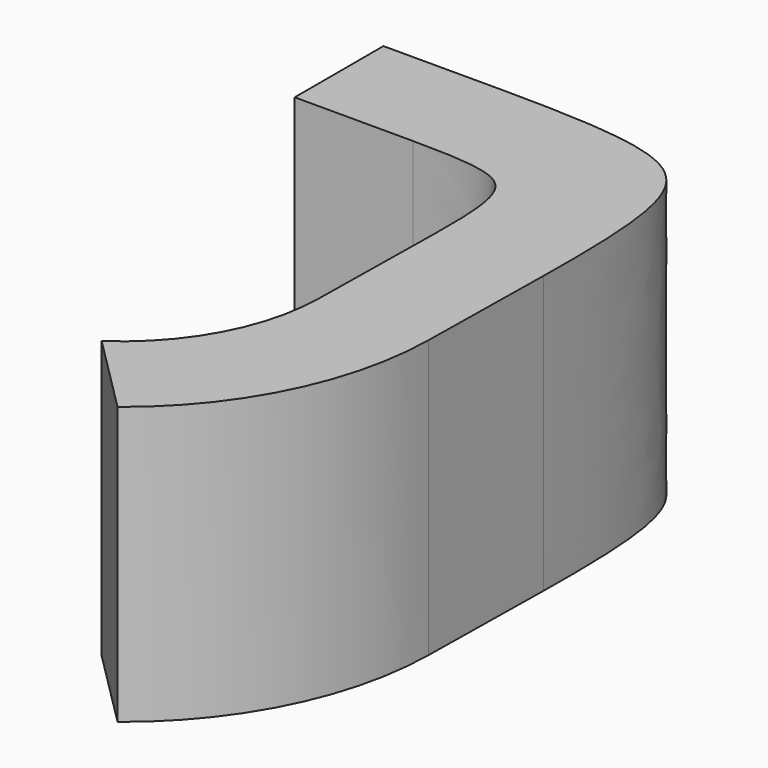
from build123d import *

# Parameters (mm, degrees)
F3_DEPTH    = 5
F4_T1_DEPTH = 5
F5_T1_DEPTH = 25.3094755674


# Not quite as in the source:
# - a fillet or chamfer that OpenCascade refuses, or shapes differently, is made with other operations: its cross-section is extruded or revolved along the edge and cut away or added
# - a feature of the source that left no trace in its solid (it failed there, or was rolled back) is left out


with BuildPart() as f3:
    # F2 (on Top) → F3 (new body)
    with BuildSketch(Plane.XY):
        with BuildLine():
            Line((5.5017601699, 0), (5.5017601699, -2))
            Line((5.5017601699, -2), (9.6698484997, -2))
            Line((9.6698484997, -2), (9.5995756294, -6.5762830432))
            ThreePointArc((9.5995756294, -6.5762830432), (9.167895168, -8.2311078505), (8.0212889249, -9.5))
            Line((8.0212889249, -9.5), (9.4518866721, -10.9305977473))
            ThreePointArc((9.4518866721, -10.9305977473), (11.0154330705, -9.0120786534), (11.5993398679, -6.6069911903))
            Line((11.5993398679, -6.6069911903), (11.7007960564, 0))
            Line((11.7007960564, 0), (5.5017601699, 0))
        make_face()
    extrude(amount=F3_DEPTH)

    # F4: fillet of radius 2 on 1 edges, made by hand

    # F4_s2 → F4_t1 (join)
    with BuildSketch(Plane.XY):
        with BuildLine():
            add(Edge.make_bspline(
                [(7.638900943, -2), (9.6698484997, -2), (9.6386651815, -4.0307081471)],
                knots=[0, 0, 0, 1, 1, 1], degree=2, weights=[1, 2.3333333333, 1]))
            Line((9.6386651815, -4.0307081471), (9.6698484997, -2))
            Line((9.6698484997, -2), (7.638900943, -2))
        make_face()
    extrude(amount=F4_T1_DEPTH)

    # F5: fillet of radius 4 on 1 edges, made by hand

    # F5_s2 → F5_t1 (cut)
    with BuildSketch(Plane.XY.offset(-10.1547377837)):
        with BuildLine():
            add(Edge.make_bspline(
                [(11.63842942, -4.0614162943), (11.7007960564, 0), (7.638900943, 0)],
                knots=[0, 0, 0, 1, 1, 1], degree=2, weights=[1, 2.3333333333, 1]))
            Line((7.638900943, 0), (11.7007960564, 0))
            Line((11.7007960564, 0), (11.63842942, -4.0614162943))
        make_face()
    extrude(amount=F5_T1_DEPTH, mode=Mode.SUBTRACT)


solid = f3.part
